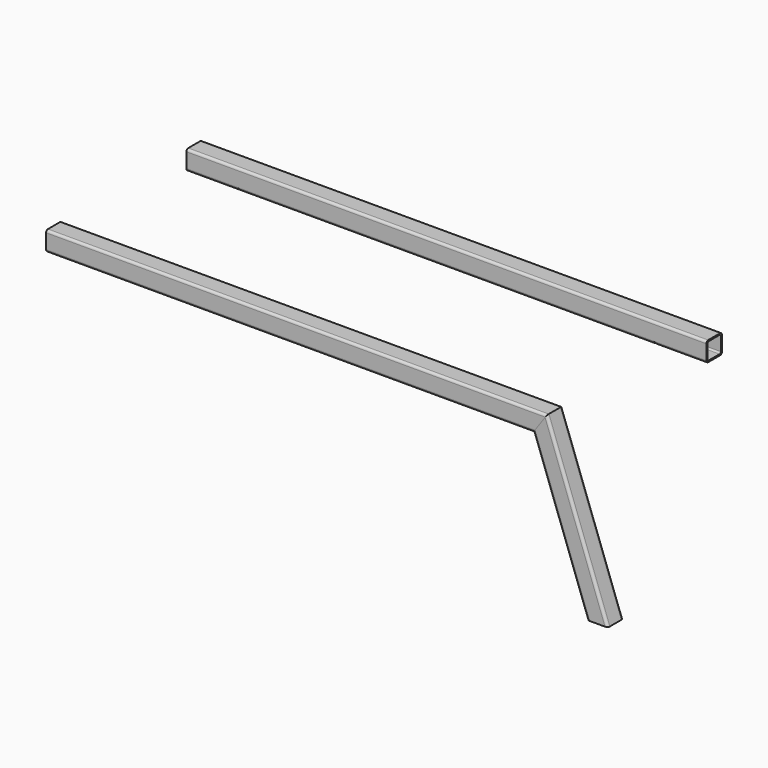
from build123d import *

# Parameters (mm, degrees)
F1_DEPTH      = 1016
F6_R          = 2.38125
F7_DEPTH      = 25.4
F7_DEPTH_BACK = 25.4
F9_DEPTH      = 50.8
F10_DEPTH     = 50.8
F13_REACH     = 736.6402660348
F15_DEPTH     = 50.8


with BuildPart() as f1:
    # F0 (on Right) → F1 (new body)
    with BuildSketch(Plane.YZ):
        with BuildLine():
            ThreePointArc((0, 4.572), (1.3391077964, 1.3391077964), (4.572, 0))
            Line((4.572, 0), (33.528, 0))
            ThreePointArc((33.528, 0), (36.7608922036, 1.3391077964), (38.1, 4.572))
            Line((38.1, 4.572), (38.1, 33.528))
            ThreePointArc((38.1, 33.528), (36.7608922036, 36.7608922036), (33.528, 38.1))
            Line((33.528, 38.1), (4.572, 38.1))
            ThreePointArc((4.572, 38.1), (1.3391077964, 36.7608922036), (0, 33.528))
            Line((0, 33.528), (0, 4.572))
        make_face()
        with BuildLine():
            ThreePointArc((2.54, 32.512), (3.4327385309, 34.6672614691), (5.588, 35.56))
            Line((5.588, 35.56), (32.512, 35.56))
            ThreePointArc((32.512, 35.56), (34.6672614691, 34.6672614691), (35.56, 32.512))
            Line((35.56, 32.512), (35.56, 5.588))
            ThreePointArc((35.56, 5.588), (34.6672614691, 3.4327385309), (32.512, 2.54))
            Line((32.512, 2.54), (5.588, 2.54))
            ThreePointArc((5.588, 2.54), (3.4327385309, 3.4327385309), (2.54, 5.588))
            Line((2.54, 5.588), (2.54, 32.512))
        make_face(mode=Mode.SUBTRACT)
    extrude(amount=F1_DEPTH)


with BuildPart() as f3_1:
    # F3: instance of F1
    add(f1.part.mirror(Plane.XZ.offset(152.4)))

    # F8 (on face) → F9 (cut)
    with BuildSketch(Plane.XZ.offset(342.9)):
        Polygon((978.7288841391, 38.1), (952.0509769333, 0), (947.5085139275, -15.6161198393), (957.4878247443, -14.9376165936), (997.0538689515, -12.2474819838), (1035.239190855, -9.6512240536), (1040.9219264984, 51.4345876873), (1012.4167203903, 54.0863908827), align=None)
    extrude(amount=-F9_DEPTH, mode=Mode.SUBTRACT)


with BuildPart() as f1_1:
    add(f1.part)

    # F6 (on 3pt) → F7 (cut, two sides)
    with BuildSketch(Plane(origin=(0, 2.286, 2.286), x_dir=(1, 0, 0), z_dir=(0, 0.7071067812, 0.7071067812))) as f7_sk:
        with Locations((914.4, 0)):
            Circle(F6_R)
        with Locations((101.6, 0)):
            Circle(F6_R)
    extrude(amount=-F7_DEPTH, mode=Mode.SUBTRACT)
    extrude(f7_sk.sketch, amount=F7_DEPTH_BACK, mode=Mode.SUBTRACT)

    # F8 (on face) → F10 (cut)
    with BuildSketch(Plane.XZ.offset(342.9)):
        Polygon((978.7288841391, 38.1), (952.0509769333, 0), (947.5085139275, -15.6161198393), (957.4878247443, -14.9376165936), (997.0538689515, -12.2474819838), (1035.239190855, -9.6512240536), (1040.9219264984, 51.4345876873), (1012.4167203903, 54.0863908827), align=None)
    extrude(amount=-F10_DEPTH, mode=Mode.SUBTRACT)


with BuildPart() as f13:
    f13_end = Plane(origin=(965.3899305362, -323.85, 19.05), x_dir=(0.5735764364, 0, 0.8191520443), z_dir=(0.8191520443, 0, -0.5735764364))
    # F12 (on line) → F13 (new body, up to a plane its end follows)
    with BuildSketch(Plane(origin=(221.2717924585, 0, -607.9392533421), x_dir=(0.9396926208, 0, 0.3420201433), z_dir=(-0.3420201433, 0, 0.9396926208))):
        with BuildLine():
            ThreePointArc((927.6552776362, -342.9), (931.2473800847, -341.4121024484), (932.7352776362, -337.82))
            Line((932.7352776362, -337.82), (932.7352776362, -309.88))
            ThreePointArc((932.7352776362, -309.88), (931.2473800847, -306.2878975516), (927.6552776362, -304.8))
            Line((927.6552776362, -304.8), (899.7152776362, -304.8))
            ThreePointArc((899.7152776362, -304.8), (896.1231751878, -306.2878975516), (894.6352776362, -309.88))
            Line((894.6352776362, -309.88), (894.6352776362, -337.82))
            ThreePointArc((894.6352776362, -337.82), (896.1231751878, -341.4121024484), (899.7152776362, -342.9))
            Line((899.7152776362, -342.9), (927.6552776362, -342.9))
        make_face()
    f13_long = extrude(amount=F13_REACH, mode=Mode.PRIVATE)
    add(split(f13_long, bisect_by=f13_end, keep=Keep.TOP, mode=Mode.PRIVATE))

    # F14 (on face) → F15 (cut)
    with BuildSketch(Plane.XZ.offset(342.9)):
        Polygon((1097.75625, -288.925), (1018.38125, -288.925), (1040.6295061111, -307.8373670578), (1091.3935899734, -315.6994581223), align=None)
    extrude(amount=-F15_DEPTH, mode=Mode.SUBTRACT)


solid = Compound([f3_1.part, f1_1.part, f13.part])
